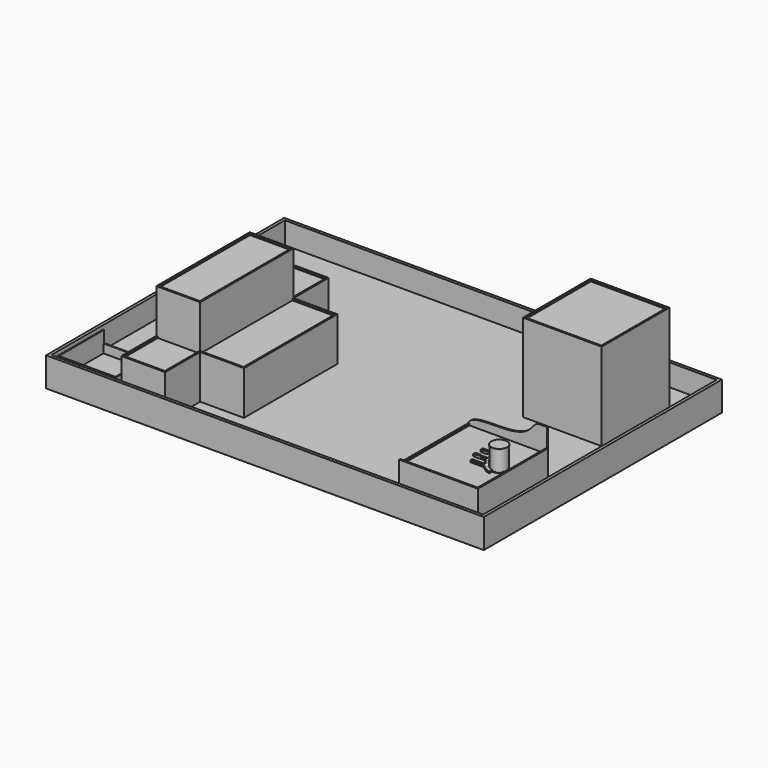
from build123d import *

# Parameters (mm, degrees)
F0_R         = 27.2
F1_DEPTH     = 2.83
F2_R         = 26.4
F3_DEPTH     = 67.36
F4_R         = 27.2
F5_DEPTH     = 2.83
F9_W         = 270
F9_H         = 300
F10_DEPTH    = 72
F12_DEPTH    = 15
F14_DEPTH    = 5
F15_W        = 5
F15_H        = 290
F16_DEPTH    = 5
F17_W        = 1500
F17_H        = 1020
F18_DEPTH    = 25
F19_W        = 270
F19_H        = 290
F20_DEPTH    = 300
F21_W        = 260
F21_H        = 280
F22_DEPTH    = 5
F23_W        = 1500
F23_H        = 1020
F23_W_2      = 1480
F23_H_2      = 1000
F24_DEPTH    = 75
F26_DEPTH    = 150
F27_W        = 150
F27_H        = 400
F28_DEPTH    = 150
F29_W        = 140
F29_H        = 390
F30_DEPTH    = 5
F31_W        = 140
F31_H        = 145
F31_W_2      = 145
F31_H_2      = 390
F32_DEPTH    = 5
F33_R        = 3
F34_DEPTH    = 4
F35_R        = 3.99999
F35_2_R      = 3.99999
F36_R        = 3
F37_DEPTH    = 8
F38_R        = 3
F39_DEPTH    = 8
F40_R        = 3
F40_R_2      = 2.5
F41_DEPTH    = 3
F42_R        = 3
F42_R_2      = 2.5
F43_DEPTH    = 3
F45_DEPTH    = 270.001
F46_W        = 200
F46_H        = 200
F46_W_2      = 194
F46_H_2      = 191
F47_DEPTH    = 30
F49_DEPTH    = 40
F50_R        = 2.5
F51_DEPTH    = 25
F52_W        = 101.480065845
F52_H        = 93.4004448354
F52_W_2      = 14.8665066808
F52_H_2      = 27.6323109865
F53_DEPTH    = 19
F54_F1_R     = 5
F54_T2_DEPTH = 37.1516298036
F54_T4_DEPTH = 52.6323109865
F54_T6_DEPTH = 37.1335703673


# Not quite as in the source:
# - a fillet or chamfer that OpenCascade refuses, or shapes differently, is made with other operations: its cross-section is extruded or revolved along the edge and cut away or added
# - a fillet or chamfer is up to 0.001 mm smaller than in the source, because OpenCascade refuses the exact size
# - a feature names something its author has since deleted; it is built from what else it names


with BuildPart() as f1:
    # F0 (on Top) → F1 (new body)
    with BuildSketch(Plane.XY):
        Circle(F0_R)
    extrude(amount=F1_DEPTH)

    # F2 (on face) → F3 (join)
    with BuildSketch(Plane.XY.offset(2.83)):
        Circle(F2_R)
    extrude(amount=F3_DEPTH)

    # F4 (on face) → F5 (join)
    with BuildSketch(Plane.XY.offset(70.19)):
        Circle(F4_R)
    extrude(amount=F5_DEPTH)


with BuildPart() as f10:
    # F9 (on Top) → F10 (new body)
    with BuildSketch(Plane.XY):
        with Locations((-87.8, 0)):
            Rectangle(F9_W, F9_H)
    extrude(amount=-F10_DEPTH)

    # F11 (on face) → F12 (join)
    with BuildSketch(Plane.XY):
        Polygon((-222.8, -145), (-222.8, -150), (47.2, -150), (47.2, 150), (42.2, 150), (42.2, -145), align=None)
    extrude(amount=F12_DEPTH)

    # F13 (on face) → F14 (join)
    with BuildSketch(Plane(origin=(0, 150, 0), x_dir=(-1, 0, 0), z_dir=(0, 1, 0))):
        with BuildLine():
            Line((-21.3134280931, 81.3575685024), (-47.2, 81.3575685024))
            Line((-47.2, 81.3575685024), (-47.2, -72))
            Line((-47.2, -72), (222.8, -72))
            Line((222.8, -72), (222.8, 0))
            add(Edge.make_bspline(
                [(-21.3134280931, 81.3575685024), (-6.3059147253, 81.3822787863), (12.9585432644, 38.1268753575), (103.6097013063, 23.6068887567), (223.0224295336, 30.7718731823), (222.8, 0)],
                knots=[0, 0, 0, 0, 0.2487100673, 0.6151112321, 1, 1, 1, 1], degree=3))
        make_face()
    extrude(amount=-F14_DEPTH)

    # F15 (on face) → F16 (join)
    with BuildSketch(Plane.XY):
        with Locations((-220.3, 0)):
            Rectangle(F15_W, F15_H)
    extrude(amount=F16_DEPTH)

    # F17 (on face) → F18 (join)
    with BuildSketch(Plane(origin=(0, 0, -72), x_dir=(1, 0, 0), z_dir=(0, 0, -1))):
        with Locations((-602.8, -260)):
            Rectangle(F17_W, F17_H)
    extrude(amount=F18_DEPTH)

    # F19 (on face) → F20 (join)
    with BuildSketch(Plane.XY.offset(-72)):
        with Locations((-87.8, 525)):
            Rectangle(F19_W, F19_H)
    extrude(amount=F20_DEPTH)

    # F21 (on face) → F22 (cut)
    with BuildSketch(Plane.XY.offset(228)):
        with Locations((-87.8, 525)):
            Rectangle(F21_W, F21_H)
    extrude(amount=-F22_DEPTH, mode=Mode.SUBTRACT)

    # F23 (on face) → F24 (join)
    with BuildSketch(Plane.XY.offset(-72)):
        with Locations((-602.8, 260)):
            Rectangle(F23_W, F23_H)
        with Locations((-602.8, 260)):
            Rectangle(F23_W_2, F23_H_2, mode=Mode.SUBTRACT)
    extrude(amount=F24_DEPTH)

    # F25 (on face) → F26 (join)
    with BuildSketch(Plane.XY.offset(-72)):
        Polygon((-952.8, 460), (-1102.8, 460), (-1102.8, -240), (-952.8, -240), (-952.8, -90), (-802.8, -90), (-802.8, 310), (-952.8, 310), align=None)
    extrude(amount=F26_DEPTH)

    # F27 (on face) → F28 (join)
    with BuildSketch(Plane.XY.offset(78)):
        with Locations((-1027.8, 110)):
            Rectangle(F27_W, F27_H)
    extrude(amount=F28_DEPTH)

    # F29 (on face) → F30 (cut)
    with BuildSketch(Plane.XY.offset(228)):
        with Locations((-1027.8, 110)):
            Rectangle(F29_W, F29_H)
    extrude(amount=-F30_DEPTH, mode=Mode.SUBTRACT)

    # F31 (on face) → F32 (cut)
    with BuildSketch(Plane.XY.offset(78)):
        with Locations((-1027.8, 382.5)):
            Rectangle(F31_W, F31_H)
        with Locations((-880.3, 110)):
            Rectangle(F31_W_2, F31_H_2)
        with Locations((-1027.8, -162.5)):
            Rectangle(F31_W, F31_H)
    extrude(amount=-F32_DEPTH, mode=Mode.SUBTRACT)

    # F46 (on face) → F47 (join)
    with BuildSketch(Plane.XY.offset(-72)):
        with Locations((-1232.8, -130)):
            Rectangle(F46_W, F46_H)
        with Locations((-1232.8, -128.5)):
            Rectangle(F46_W_2, F46_H_2, mode=Mode.SUBTRACT)
    extrude(amount=F47_DEPTH)

    # F48 (on face) → F49 (join)
    with BuildSketch(Plane.XY.offset(-42)):
        Polygon((-1329.8, -30), (-1332.8, -30), (-1332.8, -230), (-1329.8, -230), (-1135.8, -230), (-1132.8, -230), (-1132.8, -30), (-1135.8, -30), (-1135.8, -224), (-1329.8, -224), align=None)
    extrude(amount=F49_DEPTH)


with BuildPart() as f34:
    # F33 (on offset) → F34 (new body, symmetric)
    with BuildSketch(Plane.XY.offset(25)):
        with BuildLine():
            Line((-55, -12), (-74.5, -12))
            Line((-74.5, -12), (-74.5, -13))
            Line((-74.5, -13), (-65.6457513111, -13))
            ThreePointArc((-65.6457513111, -13), (-67, -16), (-65.6457513111, -19))
            Line((-65.6457513111, -19), (-74.5, -19))
            Line((-74.5, -19), (-74.5, -20))
            Line((-74.5, -20), (-55, -20))
            ThreePointArc((-55, -20), (-51, -16), (-55, -12))
        make_face()
        with Locations((-63, -16)):
            Circle(F33_R, mode=Mode.SUBTRACT)
        with Locations((-55, -16)):
            Circle(F33_R, mode=Mode.SUBTRACT)
    extrude(amount=F34_DEPTH, both=True)

    # F35 (radius 4 in the source; OpenCascade refuses exactly that, so slightly less here)
    f35_edges = [f34.edges().sort_by_distance(p)[0] for p in [
        (-74.5, -19.5, 29),
        (-74.5, -12.5, 29),
        (-74.5, -19.5, 21),
        (-74.5, -12.5, 21),
    ]]
    fillet(f35_edges, radius=F35_R)

    # F36 (on face) → F37 (join, through all)
    with BuildSketch(Plane.XZ.offset(20)):
        with Locations((-70.5, 25)):
            Circle(F36_R)
    extrude(amount=-F37_DEPTH)

    # F42 (on offset) → F43 (join, symmetric)
    with BuildSketch(Plane.XY.offset(25)):
        with Locations((-63, -16)):
            Circle(F42_R)
        with Locations((-63, -16)):
            Circle(F42_R_2, mode=Mode.SUBTRACT)
        with Locations((-55, -16)):
            Circle(F42_R)
        with Locations((-55, -16)):
            Circle(F42_R_2, mode=Mode.SUBTRACT)
    extrude(amount=F43_DEPTH, both=True)


with BuildPart() as f34b:
    # F33 (on offset) → F34, piece 2 (new body, symmetric)
    with BuildSketch(Plane.XY.offset(25)):
        with BuildLine():
            Line((-74.5, 13), (-74.5, 12))
            Line((-74.5, 12), (-55, 12))
            ThreePointArc((-55, 12), (-51, 16), (-55, 20))
            Line((-55, 20), (-74.5, 20))
            Line((-74.5, 20), (-74.5, 19))
            Line((-74.5, 19), (-65.6457513111, 19))
            ThreePointArc((-65.6457513111, 19), (-67, 16), (-65.6457513111, 13))
            Line((-65.6457513111, 13), (-74.5, 13))
        make_face()
        with Locations((-63, 16)):
            Circle(F33_R, mode=Mode.SUBTRACT)
        with Locations((-55, 16)):
            Circle(F33_R, mode=Mode.SUBTRACT)
    extrude(amount=F34_DEPTH, both=True)

    # F35#2 (radius 4 in the source; OpenCascade refuses exactly that, so slightly less here)
    f35_2_edges = [f34b.edges().sort_by_distance(p)[0] for p in [
        (-74.5, 12.5, 29),
        (-74.5, 19.5, 29),
        (-74.5, 19.5, 21),
        (-74.5, 12.5, 21),
    ]]
    fillet(f35_2_edges, radius=F35_2_R)

    # F38 (on face) → F39 (join, through all)
    with BuildSketch(Plane(origin=(0, 20, 0), x_dir=(-1, 0, 0), z_dir=(0, 1, 0))):
        with Locations((70.5, 25)):
            Circle(F38_R)
    extrude(amount=-F39_DEPTH)

    # F40 (on offset) → F41 (join, symmetric)
    with BuildSketch(Plane.XY.offset(25)):
        with Locations((-55, 16)):
            Circle(F40_R)
        with Locations((-55, 16)):
            Circle(F40_R_2, mode=Mode.SUBTRACT)
        with Locations((-63, 16)):
            Circle(F40_R)
        with Locations((-63, 16)):
            Circle(F40_R_2, mode=Mode.SUBTRACT)
    extrude(amount=F41_DEPTH, both=True)


with BuildPart() as f45_tool:
    # F44 (on face) → F45 (new body, through all)
    with BuildSketch(Plane(origin=(0, 20, 0), x_dir=(-1, 0, 0), z_dir=(0, 1, 0))):
        with BuildLine():
            Line((71.5, 26), (71.5, 27.2912878475))
            ThreePointArc((71.5, 27.2912878475), (70.5, 27.5), (69.5, 27.2912878475))
            Line((69.5, 27.2912878475), (69.5, 26))
            Line((69.5, 26), (68.2087121525, 26))
            ThreePointArc((68.2087121525, 26), (68, 25), (68.2087121525, 24))
            Line((68.2087121525, 24), (69.5, 24))
            Line((69.5, 24), (69.5, 22.7087121525))
            ThreePointArc((69.5, 22.7087121525), (70.5, 22.5), (71.5, 22.7087121525))
            Line((71.5, 22.7087121525), (71.5, 24))
            Line((71.5, 24), (72.7912878475, 24))
            ThreePointArc((72.7912878475, 24), (73, 25), (72.7912878475, 26))
            Line((72.7912878475, 26), (71.5, 26))
        make_face()
    extrude(amount=-F45_DEPTH)


with BuildPart() as f34_1:
    add(f34.part)

    # F45: cut by f45_tool
    add(f45_tool.part, mode=Mode.SUBTRACT)


with BuildPart() as f34b_1:
    add(f34b.part)

    # F45: cut by f45_tool
    add(f45_tool.part, mode=Mode.SUBTRACT)


with BuildPart() as f51:
    # F50 (on face) → F51 (new body)
    with BuildSketch(Plane.XY):
        with BuildLine():
            add(Edge.make_bspline(
                [(-46.7228069901, 20), (-30.8616701514, 18.9528241754), (-20.7438562065, 38.9112494886), (-2.8644339181, 38.4954474866)],
                knots=[0, 0, 0, 0, 47.5987233679, 47.5987233679, 47.5987233679, 47.5987233679], degree=3))
            Line((-46.7228069901, 20), (-82.8528106213, 20))
            Line((-82.8528106213, 20), (-82.8528106213, 12))
            Line((-82.8528106213, 12), (-45.5552316225, 12))
            Line((-45.5552316225, 12), (-45.5552316225, -12))
            Line((-45.5552316225, -12), (-82.8528106213, -12))
            Line((-82.8528106213, -12), (-82.8528106213, -20))
            Line((-82.8528106213, -20), (-46.7228069901, -20))
            add(Edge.make_bspline(
                [(-46.7228069901, -20), (-30.8616701514, -18.9528241754), (-20.7438562065, -38.9112494886), (-2.8644339181, -38.4954474866)],
                knots=[0, 0, 0, 0, 47.5987233679, 47.5987233679, 47.5987233679, 47.5987233679], degree=3))
            Line((-2.8644339181, -38.4954474866), (-2.8644339181, -27.0487526206))
            ThreePointArc((-2.8644339181, -27.0487526206), (-18.2777725774, -20.1435604998), (-26.6439338235, -5.4718178339))
            Line((-26.6439338235, -5.4718178339), (-26.8217978983, -5.4900531666))
            Line((-26.8217978983, -5.4900531666), (-31.7957253432, -6))
            Line((-31.7957253432, -6), (-31.7957253432, 0))
            Line((-31.7957253432, 0), (-31.7957253432, 6))
            Line((-31.7957253432, 6), (-26.8217978983, 5.4900531666))
            Line((-26.8217978983, 5.4900531666), (-26.6439338235, 5.4718178339))
            ThreePointArc((-26.6439338235, 5.4718178339), (-18.2777725774, 20.1435604998), (-2.8644339181, 27.0487526206))
            Line((-2.8644339181, 27.0487526206), (-2.8644339181, 38.4954474866))
        make_face()
        with Locations((-63, -16)):
            Circle(F50_R, mode=Mode.SUBTRACT)
        with Locations((-55, -16)):
            Circle(F50_R, mode=Mode.SUBTRACT)
        with Locations((-63, 16)):
            Circle(F50_R, mode=Mode.SUBTRACT)
        with Locations((-55, 16)):
            Circle(F50_R, mode=Mode.SUBTRACT)
    extrude(amount=F51_DEPTH)

    # F52 (on face) → F53 (cut)
    with BuildSketch(Plane.XY.offset(25)):
        with Locations((-36.2187256105, 1.0350365192)):
            Rectangle(F52_W, F52_H)
        with Locations((-28.1391041353, -0.0153128058)):
            Rectangle(F52_W_2, F52_H_2, mode=Mode.SUBTRACT)
    extrude(amount=-F53_DEPTH, mode=Mode.SUBTRACT)

    # F54: fillet of radius 5 on 6 edges, made by hand

    # F54_f1
    f54_f1_edges = [f51.edges().sort_by_distance(p)[0] for p in [
        (-29.5055722921, 13.8008426875, 6),
        (-35.5723574758, -0.0153128058, 6),
        (-29.496542574, -13.831468299, 6),
    ]]
    fillet(f54_f1_edges, radius=F54_F1_R)

    # F54_s3 → F54_t2 (cut)
    with BuildSketch(Plane.YZ.offset(-48.0723574758)):
        with BuildLine():
            ThreePointArc((-8.831468299, 25), (-12.367002205, 23.5355339059), (-13.831468299, 20))
            Line((-13.831468299, 20), (-13.931468299, 20))
            Line((-13.931468299, 20), (-13.931468299, 25.1))
            Line((-13.931468299, 25.1), (-8.831468299, 25.1))
            Line((-8.831468299, 25.1), (-8.831468299, 25))
        make_face()
    extrude(amount=F54_T2_DEPTH, mode=Mode.SUBTRACT)

    # F54_s5 → F54_t4 (cut)
    with BuildSketch(Plane.XZ.offset(-26.3008426875)):
        with BuildLine():
            ThreePointArc((-30.5723574758, 25), (-34.1078913817, 23.5355339059), (-35.5723574758, 20))
            Line((-35.5723574758, 20), (-35.6723574758, 20))
            Line((-35.6723574758, 20), (-35.6723574758, 25.1))
            Line((-35.6723574758, 25.1), (-30.5723574758, 25.1))
            Line((-30.5723574758, 25.1), (-30.5723574758, 25))
        make_face()
    extrude(amount=F54_T4_DEPTH, mode=Mode.SUBTRACT)

    # F54_s7 → F54_t6 (cut)
    with BuildSketch(Plane.YZ.offset(-48.0723574758)):
        with BuildLine():
            ThreePointArc((13.8008426875, 20), (12.3363765934, 23.5355339059), (8.8008426875, 25))
            Line((8.8008426875, 25), (8.8008426875, 25.1))
            Line((8.8008426875, 25.1), (13.9008426875, 25.1))
            Line((13.9008426875, 25.1), (13.9008426875, 20))
            Line((13.9008426875, 20), (13.8008426875, 20))
        make_face()
    extrude(amount=F54_T6_DEPTH, mode=Mode.SUBTRACT)


solid = Compound([f1.part, f10.part, f34_1.part, f34b_1.part, f51.part])
